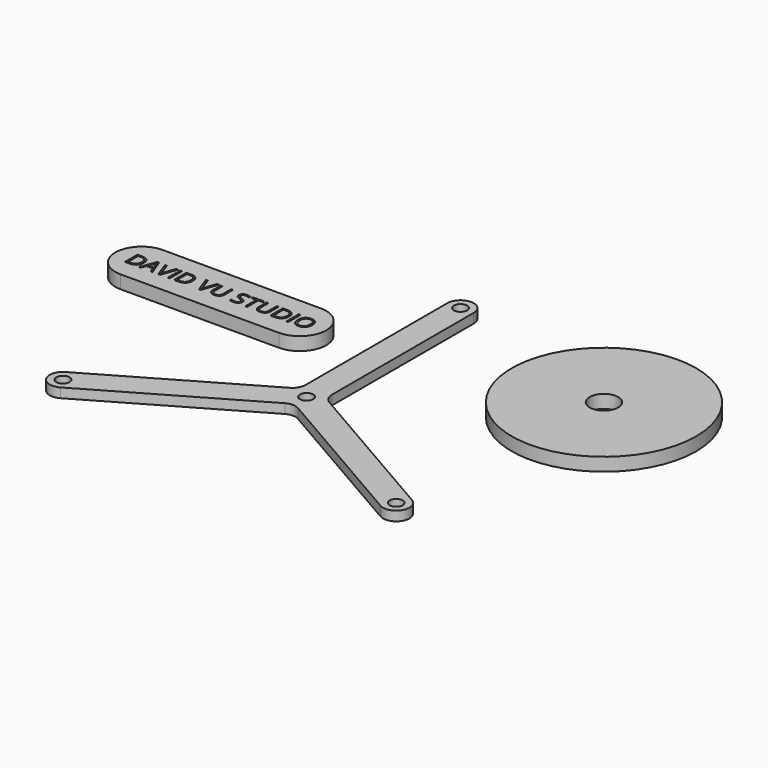
from build123d import *

# Parameters (mm, degrees)
F0_R     = 1.5875
F1_DEPTH = 2.286
F0_R_2   = 22.225
F0_R_3   = 3.429
F2_DEPTH = 3.175
F0_W     = 0.4375697521
F0_H     = 3.7650775848
F3_DEPTH = 3.175


with BuildPart() as f1:
    # F0 (on Top) → F1 (new body)
    with BuildSketch(Plane.XY):
        with BuildLine():
            Line((0, 46.355), (0, 3.6661742094))
            ThreePointArc((0, 3.6661742094), (-0.425369343, 2.0786742094), (-1.5875, 0.9165435523))
            Line((-1.5875, 0.9165435523), (-38.5571075924, -20.427869343))
            ThreePointArc((-38.5571075924, -20.427869343), (-39.7192382494, -24.765), (-35.3821075924, -25.927130657))
            Line((-35.3821075924, -25.927130657), (1.5875, -4.5827177617))
            ThreePointArc((1.5875, -4.5827177617), (3.175, -4.1573484187), (4.7625, -4.5827177617))
            Line((4.7625, -4.5827177617), (41.7321075924, -25.927130657))
            ThreePointArc((41.7321075924, -25.927130657), (46.0692382494, -24.765), (44.9071075924, -20.427869343))
            Line((44.9071075924, -20.427869343), (7.9375, 0.9165435523))
            ThreePointArc((7.9375, 0.9165435523), (6.775369343, 2.0786742094), (6.35, 3.6661742094))
            Line((6.35, 3.6661742094), (6.35, 46.355))
            ThreePointArc((6.35, 46.355), (3.175, 49.53), (0, 46.355))
        make_face()
        with Locations((-36.9696075924, -23.1775)):
            Circle(F0_R, mode=Mode.SUBTRACT)
        with Locations((3.175, 0)):
            Circle(F0_R, mode=Mode.SUBTRACT)
        with Locations((43.3196075924, -23.1775)):
            Circle(F0_R, mode=Mode.SUBTRACT)
        with Locations((3.175, 46.355)):
            Circle(F0_R, mode=Mode.SUBTRACT)
    extrude(amount=F1_DEPTH)


with BuildPart() as f2:
    # F0 (on Top) → F2 (new body)
    with BuildSketch(Plane.XY):
        with Locations((49.2994225452, 31.8949542811)):
            Circle(F0_R_2)
        with Locations((49.2994225452, 31.8949542811)):
            Circle(F0_R_3, mode=Mode.SUBTRACT)
    extrude(amount=F2_DEPTH)


with BuildPart() as f3:
    # F0 (on Top) → F3 (new body)
    with BuildSketch(Plane.XY):
        with BuildLine():
            ThreePointArc((-54.2539432645, 28.4871041447), (-60.6039432645, 22.1371041447), (-54.2539432645, 15.7871041447))
            Line((-54.2539432645, 15.7871041447), (-16.1539432645, 15.7871041447))
            ThreePointArc((-16.1539432645, 15.7871041447), (-9.8039432645, 22.1371041447), (-16.1539432645, 28.4871041447))
            Line((-16.1539432645, 28.4871041447), (-54.2539432645, 28.4871041447))
        make_face()
        with BuildLine():
            add(Edge.make_bspline(
                [(-54.2622953035, 23.5449205843), (-53.7756946657, 23.0583199466), (-53.7756946657, 22.1848285393)],
                knots=[0, 0, 0, 1, 1, 1], degree=2))
            add(Edge.make_bspline(
                [(-53.7756946657, 22.1848285393), (-53.7756946657, 21.2528296887), (-54.2816604432, 20.759636663)],
                knots=[0, 0, 0, 1, 1, 1], degree=2))
            add(Edge.make_bspline(
                [(-54.2816604432, 20.759636663), (-54.7876262206, 20.2664436373), (-55.7377541381, 20.2664436373)],
                knots=[0, 0, 0, 1, 1, 1], degree=2))
            Line((-55.7377541381, 20.2664436373), (-56.7809995359, 20.2664436373))
            Line((-56.7809995359, 20.2664436373), (-56.7809995359, 24.0315212221))
            Line((-56.7809995359, 24.0315212221), (-55.6273316395, 24.0315212221))
            add(Edge.make_bspline(
                [(-55.6273316395, 24.0315212221), (-54.7488959412, 24.0315212221), (-54.2622953035, 23.5449205843)],
                knots=[0, 0, 0, 1, 1, 1], degree=2))
        make_face(mode=Mode.SUBTRACT)
        Polygon((-50.1160952886, 20.2664436373), (-50.5693219622, 20.2664436373), (-51.0382055573, 21.4637861041), (-52.5470383561, 21.4637861041), (-53.0101536116, 20.2664436373), (-53.4534917032, 20.2664436373), (-51.9652601169, 24.0471781435), (-51.5969104385, 24.0471781435), align=None, mode=Mode.SUBTRACT)
        with BuildLine():
            Line((-48.3081328853, 21.6104667366), (-47.447826254, 24.0315212221))
            Line((-47.447826254, 24.0315212221), (-46.9772945619, 24.0315212221))
            Line((-46.9772945619, 24.0315212221), (-48.3336783887, 20.2664436373))
            Line((-48.3336783887, 20.2664436373), (-48.7663038499, 20.2664436373))
            Line((-48.7663038499, 20.2664436373), (-50.1160952886, 24.0315212221))
            Line((-50.1160952886, 24.0315212221), (-49.6521559846, 24.0315212221))
            Line((-49.6521559846, 24.0315212221), (-48.7869050623, 21.5956338637))
            add(Edge.make_bspline(
                [(-48.7869050623, 21.5956338637), (-48.6377522843, 21.17536913), (-48.5504031435, 20.7790018027)],
                knots=[0, 0, 0, 1, 1, 1], degree=2))
            add(Edge.make_bspline(
                [(-48.5504031435, 20.7790018027), (-48.4572856633, 21.1959703424), (-48.3081328853, 21.6104667366)],
                knots=[0, 0, 0, 1, 1, 1], degree=2))
        make_face(mode=Mode.SUBTRACT)
        with Locations((-46.2410072295, 22.1489824297)):
            Rectangle(F0_W, F0_H, mode=Mode.SUBTRACT)
        with BuildLine():
            add(Edge.make_bspline(
                [(-42.4709853537, 23.5449205843), (-41.984384716, 23.0583199466), (-41.984384716, 22.1848285393)],
                knots=[0, 0, 0, 1, 1, 1], degree=2))
            add(Edge.make_bspline(
                [(-41.984384716, 22.1848285393), (-41.984384716, 21.2528296887), (-42.4903504934, 20.759636663)],
                knots=[0, 0, 0, 1, 1, 1], degree=2))
            add(Edge.make_bspline(
                [(-42.4903504934, 20.759636663), (-42.9963162708, 20.2664436373), (-43.9464441884, 20.2664436373)],
                knots=[0, 0, 0, 1, 1, 1], degree=2))
            Line((-43.9464441884, 20.2664436373), (-44.9896895861, 20.2664436373))
            Line((-44.9896895861, 20.2664436373), (-44.9896895861, 24.0315212221))
            Line((-44.9896895861, 24.0315212221), (-43.8360216897, 24.0315212221))
            add(Edge.make_bspline(
                [(-43.8360216897, 24.0315212221), (-42.9575859915, 24.0315212221), (-42.4709853537, 23.5449205843)],
                knots=[0, 0, 0, 1, 1, 1], degree=2))
        make_face(mode=Mode.SUBTRACT)
        with BuildLine():
            Line((-38.4838266989, 21.6104667366), (-37.6235200676, 24.0315212221))
            Line((-37.6235200676, 24.0315212221), (-37.1529883755, 24.0315212221))
            Line((-37.1529883755, 24.0315212221), (-38.5093722023, 20.2664436373))
            Line((-38.5093722023, 20.2664436373), (-38.9419976635, 20.2664436373))
            Line((-38.9419976635, 20.2664436373), (-40.2917891023, 24.0315212221))
            Line((-40.2917891023, 24.0315212221), (-39.8278497982, 24.0315212221))
            Line((-39.8278497982, 24.0315212221), (-38.9625988759, 21.5956338637))
            add(Edge.make_bspline(
                [(-38.9625988759, 21.5956338637), (-38.8134460979, 21.17536913), (-38.7260969571, 20.7790018027)],
                knots=[0, 0, 0, 1, 1, 1], degree=2))
            add(Edge.make_bspline(
                [(-38.7260969571, 20.7790018027), (-38.6329794769, 21.1959703424), (-38.4838266989, 21.6104667366)],
                knots=[0, 0, 0, 1, 1, 1], degree=2))
        make_face(mode=Mode.SUBTRACT)
        with BuildLine():
            Line((-34.2300883551, 24.0315212221), (-33.792518603, 24.0315212221))
            Line((-33.792518603, 24.0315212221), (-33.792518603, 21.5956338637))
            add(Edge.make_bspline(
                [(-33.792518603, 21.5956338637), (-33.792518603, 20.9512279387), (-34.1814694938, 20.5828782603)],
                knots=[0, 0, 0, 1, 1, 1], degree=2))
            add(Edge.make_bspline(
                [(-34.1814694938, 20.5828782603), (-34.5704203846, 20.214528582), (-35.250260395, 20.214528582)],
                knots=[0, 0, 0, 1, 1, 1], degree=2))
            add(Edge.make_bspline(
                [(-35.250260395, 20.214528582), (-35.9301004053, 20.214528582), (-36.3021583019, 20.58576243)],
                knots=[0, 0, 0, 1, 1, 1], degree=2))
            add(Edge.make_bspline(
                [(-36.3021583019, 20.58576243), (-36.6742161985, 20.9569962781), (-36.6742161985, 21.6055224456)],
                knots=[0, 0, 0, 1, 1, 1], degree=2))
            Line((-36.6742161985, 21.6055224456), (-36.6742161985, 24.0315212221))
            Line((-36.6742161985, 24.0315212221), (-36.2358223979, 24.0315212221))
            Line((-36.2358223979, 24.0315212221), (-36.2358223979, 21.5750326512))
            add(Edge.make_bspline(
                [(-36.2358223979, 21.5750326512), (-36.2358223979, 21.1036769107), (-35.9783072424, 20.8511060462)],
                knots=[0, 0, 0, 1, 1, 1], degree=2))
            add(Edge.make_bspline(
                [(-35.9783072424, 20.8511060462), (-35.720792087, 20.5985351818), (-35.2214186976, 20.5985351818)],
                knots=[0, 0, 0, 1, 1, 1], degree=2))
            add(Edge.make_bspline(
                [(-35.2214186976, 20.5985351818), (-34.745118666, 20.5985351818), (-34.4876035106, 20.852342119)],
                knots=[0, 0, 0, 1, 1, 1], degree=2))
            add(Edge.make_bspline(
                [(-34.4876035106, 20.852342119), (-34.2300883551, 21.1061490562), (-34.2300883551, 21.5799769422)],
                knots=[0, 0, 0, 1, 1, 1], degree=2))
            Line((-34.2300883551, 21.5799769422), (-34.2300883551, 24.0315212221))
        make_face(mode=Mode.SUBTRACT)
        with BuildLine():
            add(Edge.make_bspline(
                [(-29.5239473863, 21.8964115652), (-29.301454292, 21.654141307), (-29.301454292, 21.2684866102)],
                knots=[0, 0, 0, 1, 1, 1], degree=2))
            add(Edge.make_bspline(
                [(-29.301454292, 21.2684866102), (-29.301454292, 20.7715853662), (-29.6619755096, 20.4930569741)],
                knots=[0, 0, 0, 1, 1, 1], degree=2))
            add(Edge.make_bspline(
                [(-29.6619755096, 20.4930569741), (-30.0224967273, 20.214528582), (-30.6405331003, 20.214528582)],
                knots=[0, 0, 0, 1, 1, 1], degree=2))
            add(Edge.make_bspline(
                [(-30.6405331003, 20.214528582), (-31.3096604802, 20.214528582), (-31.6705937221, 20.3875787664)],
                knots=[0, 0, 0, 1, 1, 1], degree=2))
            Line((-31.6705937221, 20.3875787664), (-31.6705937221, 20.8094915971))
            add(Edge.make_bspline(
                [(-31.6705937221, 20.8094915971), (-31.4382120458, 20.7122538744), (-31.1654519932, 20.6553945281)],
                knots=[0, 0, 0, 1, 1, 1], degree=2))
            add(Edge.make_bspline(
                [(-31.1654519932, 20.6553945281), (-30.8926919405, 20.5985351818), (-30.6248761789, 20.5985351818)],
                knots=[0, 0, 0, 1, 1, 1], degree=2))
            add(Edge.make_bspline(
                [(-30.6248761789, 20.5985351818), (-30.1873064267, 20.5985351818), (-29.9656373809, 20.764580954)],
                knots=[0, 0, 0, 1, 1, 1], degree=2))
            add(Edge.make_bspline(
                [(-29.9656373809, 20.764580954), (-29.7439683351, 20.9306267262), (-29.7439683351, 21.2272841853)],
                knots=[0, 0, 0, 1, 1, 1], degree=2))
            add(Edge.make_bspline(
                [(-29.7439683351, 21.2272841853), (-29.7439683351, 21.4225836792), (-29.8226649666, 21.5474270266)],
                knots=[0, 0, 0, 1, 1, 1], degree=2))
            add(Edge.make_bspline(
                [(-29.8226649666, 21.5474270266), (-29.9013615981, 21.6722703739), (-30.0855364373, 21.7781606058)],
                knots=[0, 0, 0, 1, 1, 1], degree=2))
            add(Edge.make_bspline(
                [(-30.0855364373, 21.7781606058), (-30.2697112765, 21.8840508378), (-30.6454773913, 22.0175466943)],
                knots=[0, 0, 0, 1, 1, 1], degree=2))
            add(Edge.make_bspline(
                [(-30.6454773913, 22.0175466943), (-31.1703962842, 22.2054297518), (-31.3957735482, 22.4629449072)],
                knots=[0, 0, 0, 1, 1, 1], degree=2))
            add(Edge.make_bspline(
                [(-31.3957735482, 22.4629449072), (-31.6211508123, 22.7204600626), (-31.6211508123, 23.1349564569)],
                knots=[0, 0, 0, 1, 1, 1], degree=2))
            add(Edge.make_bspline(
                [(-31.6211508123, 23.1349564569), (-31.6211508123, 23.5700540635), (-31.294415583, 23.8275692189)],
                knots=[0, 0, 0, 1, 1, 1], degree=2))
            add(Edge.make_bspline(
                [(-31.294415583, 23.8275692189), (-30.9676803538, 24.0850843744), (-30.4287526365, 24.0850843744)],
                knots=[0, 0, 0, 1, 1, 1], degree=2))
            add(Edge.make_bspline(
                [(-30.4287526365, 24.0850843744), (-29.8675756097, 24.0850843744), (-29.3962198692, 23.87907225)],
                knots=[0, 0, 0, 1, 1, 1], degree=2))
            Line((-29.3962198692, 23.87907225), (-29.5330119198, 23.4983618442))
            add(Edge.make_bspline(
                [(-29.5330119198, 23.4983618442), (-29.9994233693, 23.6936613381), (-30.439465267, 23.6936613381)],
                knots=[0, 0, 0, 1, 1, 1], degree=2))
            add(Edge.make_bspline(
                [(-30.439465267, 23.6936613381), (-30.7872137329, 23.6936613381), (-30.982925251, 23.5445085601)],
                knots=[0, 0, 0, 1, 1, 1], degree=2))
            add(Edge.make_bspline(
                [(-30.982925251, 23.5445085601), (-31.1786367692, 23.395355782), (-31.1786367692, 23.1300121659)],
                knots=[0, 0, 0, 1, 1, 1], degree=2))
            add(Edge.make_bspline(
                [(-31.1786367692, 23.1300121659), (-31.1786367692, 22.934712672), (-31.1065325256, 22.8094573004)],
                knots=[0, 0, 0, 1, 1, 1], degree=2))
            add(Edge.make_bspline(
                [(-31.1065325256, 22.8094573004), (-31.0344282821, 22.6842019288), (-30.8630261946, 22.5799597938)],
                knots=[0, 0, 0, 1, 1, 1], degree=2))
            add(Edge.make_bspline(
                [(-30.8630261946, 22.5799597938), (-30.6916241072, 22.4757176589), (-30.3389313503, 22.3496382388)],
                knots=[0, 0, 0, 1, 1, 1], degree=2))
            add(Edge.make_bspline(
                [(-30.3389313503, 22.3496382388), (-29.7464404806, 22.1386818235), (-29.5239473863, 21.8964115652)],
                knots=[0, 0, 0, 1, 1, 1], degree=2))
        make_face(mode=Mode.SUBTRACT)
        Polygon((-27.3723567595, 23.6425703313), (-27.3723567595, 20.2664436373), (-27.8099265116, 20.2664436373), (-27.8099265116, 23.6425703313), (-29.0023246874, 23.6425703313), (-29.0023246874, 24.0315212221), (-26.1799585837, 24.0315212221), (-26.1799585837, 23.6425703313), align=None, mode=Mode.SUBTRACT)
        with BuildLine():
            Line((-23.2076156535, 24.0315212221), (-22.7700459014, 24.0315212221))
            Line((-22.7700459014, 24.0315212221), (-22.7700459014, 21.5956338637))
            add(Edge.make_bspline(
                [(-22.7700459014, 21.5956338637), (-22.7700459014, 20.9512279387), (-23.1589967921, 20.5828782603)],
                knots=[0, 0, 0, 1, 1, 1], degree=2))
            add(Edge.make_bspline(
                [(-23.1589967921, 20.5828782603), (-23.5479476829, 20.214528582), (-24.2277876933, 20.214528582)],
                knots=[0, 0, 0, 1, 1, 1], degree=2))
            add(Edge.make_bspline(
                [(-24.2277876933, 20.214528582), (-24.9076277037, 20.214528582), (-25.2796856003, 20.58576243)],
                knots=[0, 0, 0, 1, 1, 1], degree=2))
            add(Edge.make_bspline(
                [(-25.2796856003, 20.58576243), (-25.6517434969, 20.9569962781), (-25.6517434969, 21.6055224456)],
                knots=[0, 0, 0, 1, 1, 1], degree=2))
            Line((-25.6517434969, 21.6055224456), (-25.6517434969, 24.0315212221))
            Line((-25.6517434969, 24.0315212221), (-25.2133496962, 24.0315212221))
            Line((-25.2133496962, 24.0315212221), (-25.2133496962, 21.5750326512))
            add(Edge.make_bspline(
                [(-25.2133496962, 21.5750326512), (-25.2133496962, 21.1036769107), (-24.9558345408, 20.8511060462)],
                knots=[0, 0, 0, 1, 1, 1], degree=2))
            add(Edge.make_bspline(
                [(-24.9558345408, 20.8511060462), (-24.6983193853, 20.5985351818), (-24.1989459959, 20.5985351818)],
                knots=[0, 0, 0, 1, 1, 1], degree=2))
            add(Edge.make_bspline(
                [(-24.1989459959, 20.5985351818), (-23.7226459644, 20.5985351818), (-23.4651308089, 20.852342119)],
                knots=[0, 0, 0, 1, 1, 1], degree=2))
            add(Edge.make_bspline(
                [(-23.4651308089, 20.852342119), (-23.2076156535, 21.1061490562), (-23.2076156535, 21.5799769422)],
                knots=[0, 0, 0, 1, 1, 1], degree=2))
            Line((-23.2076156535, 21.5799769422), (-23.2076156535, 24.0315212221))
        make_face(mode=Mode.SUBTRACT)
        with BuildLine():
            add(Edge.make_bspline(
                [(-19.2550670356, 23.5449205843), (-18.7684663978, 23.0583199466), (-18.7684663978, 22.1848285393)],
                knots=[0, 0, 0, 1, 1, 1], degree=2))
            add(Edge.make_bspline(
                [(-18.7684663978, 22.1848285393), (-18.7684663978, 21.2528296887), (-19.2744321752, 20.759636663)],
                knots=[0, 0, 0, 1, 1, 1], degree=2))
            add(Edge.make_bspline(
                [(-19.2744321752, 20.759636663), (-19.7803979527, 20.2664436373), (-20.7305258702, 20.2664436373)],
                knots=[0, 0, 0, 1, 1, 1], degree=2))
            Line((-20.7305258702, 20.2664436373), (-21.773771268, 20.2664436373))
            Line((-21.773771268, 20.2664436373), (-21.773771268, 24.0315212221))
            Line((-21.773771268, 24.0315212221), (-20.6201033716, 24.0315212221))
            add(Edge.make_bspline(
                [(-20.6201033716, 24.0315212221), (-19.7416676733, 24.0315212221), (-19.2550670356, 23.5449205843)],
                knots=[0, 0, 0, 1, 1, 1], degree=2))
        make_face(mode=Mode.SUBTRACT)
        with Locations((-17.7099761029, 22.1489824297)):
            Rectangle(F0_W, F0_H, mode=Mode.SUBTRACT)
        with BuildLine():
            add(Edge.make_bspline(
                [(-13.6461809378, 23.575822403), (-13.1904821187, 23.0607920921), (-13.1904821187, 22.1543387449)],
                knots=[0, 0, 0, 1, 1, 1], degree=2))
            add(Edge.make_bspline(
                [(-13.1904821187, 22.1543387449), (-13.1904821187, 21.2503575432), (-13.6478290348, 20.7324430626)],
                knots=[0, 0, 0, 1, 1, 1], degree=2))
            add(Edge.make_bspline(
                [(-13.6478290348, 20.7324430626), (-14.1051759509, 20.214528582), (-14.9185118178, 20.214528582)],
                knots=[0, 0, 0, 1, 1, 1], degree=2))
            add(Edge.make_bspline(
                [(-14.9185118178, 20.214528582), (-15.7499767517, 20.214528582), (-16.2019673526, 20.7233785291)],
                knots=[0, 0, 0, 1, 1, 1], degree=2))
            add(Edge.make_bspline(
                [(-16.2019673526, 20.7233785291), (-16.6539579534, 21.2322284763), (-16.6539579534, 22.1592830359)],
                knots=[0, 0, 0, 1, 1, 1], degree=2))
            add(Edge.make_bspline(
                [(-16.6539579534, 22.1592830359), (-16.6539579534, 23.078921159), (-16.2007312798, 23.5848869365)],
                knots=[0, 0, 0, 1, 1, 1], degree=2))
            add(Edge.make_bspline(
                [(-16.2007312798, 23.5848869365), (-15.7475046062, 24.0908527139), (-14.9135675268, 24.0908527139)],
                knots=[0, 0, 0, 1, 1, 1], degree=2))
            add(Edge.make_bspline(
                [(-14.9135675268, 24.0908527139), (-14.1018797569, 24.0908527139), (-13.6461809378, 23.575822403)],
                knots=[0, 0, 0, 1, 1, 1], degree=2))
        make_face(mode=Mode.SUBTRACT)
    extrude(amount=F3_DEPTH)


with BuildPart() as f3b:
    # F0 (on Top) → F3, piece 2 (new body)
    with BuildSketch(Plane.XY):
        with BuildLine():
            add(Edge.make_bspline(
                [(-15.8649315171, 23.3038863988), (-16.1908426979, 22.9083431201), (-16.1908426979, 22.1543387449)],
                knots=[0, 0, 0, 1, 1, 1], degree=2))
            add(Edge.make_bspline(
                [(-16.1908426979, 22.1543387449), (-16.1908426979, 21.3896217393), (-15.8649315171, 20.9940784605)],
                knots=[0, 0, 0, 1, 1, 1], degree=2))
            add(Edge.make_bspline(
                [(-15.8649315171, 20.9940784605), (-15.5390203364, 20.5985351818), (-14.9185118178, 20.5985351818)],
                knots=[0, 0, 0, 1, 1, 1], degree=2))
            add(Edge.make_bspline(
                [(-14.9185118178, 20.5985351818), (-14.2930590083, 20.5985351818), (-13.9737402155, 20.9924303635)],
                knots=[0, 0, 0, 1, 1, 1], degree=2))
            add(Edge.make_bspline(
                [(-13.9737402155, 20.9924303635), (-13.6544214228, 21.3863255453), (-13.6544214228, 22.1543387449)],
                knots=[0, 0, 0, 1, 1, 1], degree=2))
            add(Edge.make_bspline(
                [(-13.6544214228, 22.1543387449), (-13.6544214228, 22.9141114595), (-13.9725041428, 23.3067705686)],
                knots=[0, 0, 0, 1, 1, 1], degree=2))
            add(Edge.make_bspline(
                [(-13.9725041428, 23.3067705686), (-14.2905868628, 23.6994296776), (-14.9135675268, 23.6994296776)],
                knots=[0, 0, 0, 1, 1, 1], degree=2))
            add(Edge.make_bspline(
                [(-14.9135675268, 23.6994296776), (-15.5390203364, 23.6994296776), (-15.8649315171, 23.3038863988)],
                knots=[0, 0, 0, 1, 1, 1], degree=2))
        make_face()
    extrude(amount=F3_DEPTH)


with BuildPart() as f3c:
    # F0 (on Top) → F3, piece 3 (new body)
    with BuildSketch(Plane.XY):
        with BuildLine():
            add(Edge.make_bspline(
                [(-19.6258888594, 21.0299245702), (-19.2315816534, 21.4151672427), (-19.2315816534, 22.1691716179)],
                knots=[0, 0, 0, 1, 1, 1], degree=2))
            add(Edge.make_bspline(
                [(-19.2315816534, 22.1691716179), (-19.2315816534, 22.9058709746), (-19.6011674045, 23.2791649439)],
                knots=[0, 0, 0, 1, 1, 1], degree=2))
            add(Edge.make_bspline(
                [(-19.6011674045, 23.2791649439), (-19.9707531556, 23.6524589132), (-20.7000360758, 23.6524589132)],
                knots=[0, 0, 0, 1, 1, 1], degree=2))
            Line((-20.7000360758, 23.6524589132), (-21.3362015158, 23.6524589132))
            Line((-21.3362015158, 23.6524589132), (-21.3362015158, 20.6446818976))
            Line((-21.3362015158, 20.6446818976), (-20.803042138, 20.6446818976))
            add(Edge.make_bspline(
                [(-20.803042138, 20.6446818976), (-20.0201960654, 20.6446818976), (-19.6258888594, 21.0299245702)],
                knots=[0, 0, 0, 1, 1, 1], degree=2))
        make_face()
    extrude(amount=F3_DEPTH)


with BuildPart() as f3d:
    # F0 (on Top) → F3, piece 4 (new body)
    with BuildSketch(Plane.XY):
        with BuildLine():
            add(Edge.make_bspline(
                [(-42.8418071776, 21.0299245702), (-42.4474999715, 21.4151672427), (-42.4474999715, 22.1691716179)],
                knots=[0, 0, 0, 1, 1, 1], degree=2))
            add(Edge.make_bspline(
                [(-42.4474999715, 22.1691716179), (-42.4474999715, 22.9058709746), (-42.8170857226, 23.2791649439)],
                knots=[0, 0, 0, 1, 1, 1], degree=2))
            add(Edge.make_bspline(
                [(-42.8170857226, 23.2791649439), (-43.1866714737, 23.6524589132), (-43.915954394, 23.6524589132)],
                knots=[0, 0, 0, 1, 1, 1], degree=2))
            Line((-43.915954394, 23.6524589132), (-44.552119834, 23.6524589132))
            Line((-44.552119834, 23.6524589132), (-44.552119834, 20.6446818976))
            Line((-44.552119834, 20.6446818976), (-44.0189604561, 20.6446818976))
            add(Edge.make_bspline(
                [(-44.0189604561, 20.6446818976), (-43.2361143836, 20.6446818976), (-42.8418071776, 21.0299245702)],
                knots=[0, 0, 0, 1, 1, 1], degree=2))
        make_face()
    extrude(amount=F3_DEPTH)


with BuildPart() as f3e:
    # F0 (on Top) → F3, piece 5 (new body)
    with BuildSketch(Plane.XY):
        with BuildLine():
            add(Edge.make_bspline(
                [(-54.6331171273, 21.0299245702), (-54.2388099213, 21.4151672427), (-54.2388099213, 22.1691716179)],
                knots=[0, 0, 0, 1, 1, 1], degree=2))
            add(Edge.make_bspline(
                [(-54.2388099213, 22.1691716179), (-54.2388099213, 22.9058709746), (-54.6083956724, 23.2791649439)],
                knots=[0, 0, 0, 1, 1, 1], degree=2))
            add(Edge.make_bspline(
                [(-54.6083956724, 23.2791649439), (-54.9779814235, 23.6524589132), (-55.7072643437, 23.6524589132)],
                knots=[0, 0, 0, 1, 1, 1], degree=2))
            Line((-55.7072643437, 23.6524589132), (-56.3434297837, 23.6524589132))
            Line((-56.3434297837, 23.6524589132), (-56.3434297837, 20.6446818976))
            Line((-56.3434297837, 20.6446818976), (-55.8102704059, 20.6446818976))
            add(Edge.make_bspline(
                [(-55.8102704059, 20.6446818976), (-55.0274243333, 20.6446818976), (-54.6331171273, 21.0299245702)],
                knots=[0, 0, 0, 1, 1, 1], degree=2))
        make_face()
    extrude(amount=F3_DEPTH)


with BuildPart() as f3f:
    # F0 (on Top) → F3, piece 6 (new body)
    with BuildSketch(Plane.XY):
        with BuildLine():
            Line((-52.3921172386, 21.8576812858), (-51.1741735593, 21.8576812858))
            Line((-51.1741735593, 21.8576812858), (-51.61256736, 23.0245339582))
            add(Edge.make_bspline(
                [(-51.61256736, 23.0245339582), (-51.6974443552, 23.246203004), (-51.7872656414, 23.567581918)],
                knots=[0, 0, 0, 1, 1, 1], degree=2))
            add(Edge.make_bspline(
                [(-51.7872656414, 23.567581918), (-51.8441249878, 23.3203673688), (-51.9496031954, 23.0245339582)],
                knots=[0, 0, 0, 1, 1, 1], degree=2))
            Line((-51.9496031954, 23.0245339582), (-52.3921172386, 21.8576812858))
        make_face()
    extrude(amount=F3_DEPTH)


solid = Compound([f1.part, f2.part, f3.part, f3b.part, f3c.part, f3d.part, f3e.part, f3f.part])
